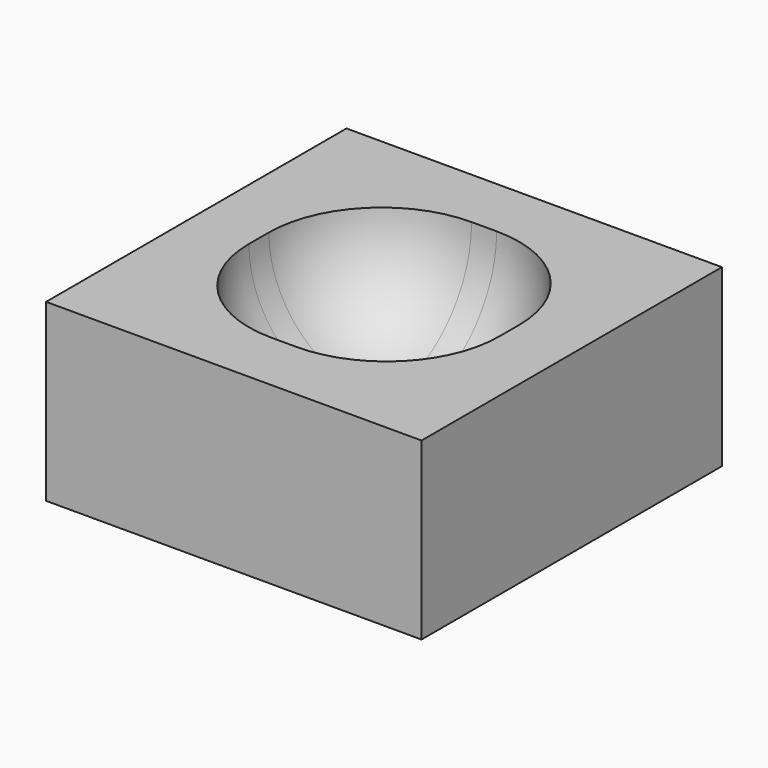
from build123d import *

# Parameters (mm, degrees)
F0_W     = 150
F0_H     = 150
F1_DEPTH = 70
F2_T     = -25
F3_R     = 44.99999


# Not quite as in the source:
# - a fillet or chamfer is up to 0.001 mm smaller than in the source, because OpenCascade refuses the exact size


with BuildPart() as f1:
    # F0 (on Top) → F1 (new body)
    with BuildSketch(Plane.XY):
        Rectangle(F0_W, F0_H)
    extrude(amount=F1_DEPTH)

    # F2
    f2_openings = [f1.faces().sort_by_distance(p)[0] for p in [
        (0, 0, 70),
    ]]
    offset(amount=F2_T, openings=f2_openings)

    # F3 (radius 45 in the source; OpenCascade refuses exactly that, so slightly less here)
    f3_edges = [f1.edges().sort_by_distance(p)[0] for p in [
        (0, 50, 25),
        (-50, 0, 25),
        (50, 0, 25),
        (0, -50, 25),
        (50, -50, 47.5),
        (50, 50, 47.5),
        (-50, 50, 47.5),
        (-50, -50, 47.5),
    ]]
    fillet(f3_edges, radius=F3_R)


solid = f1.part
